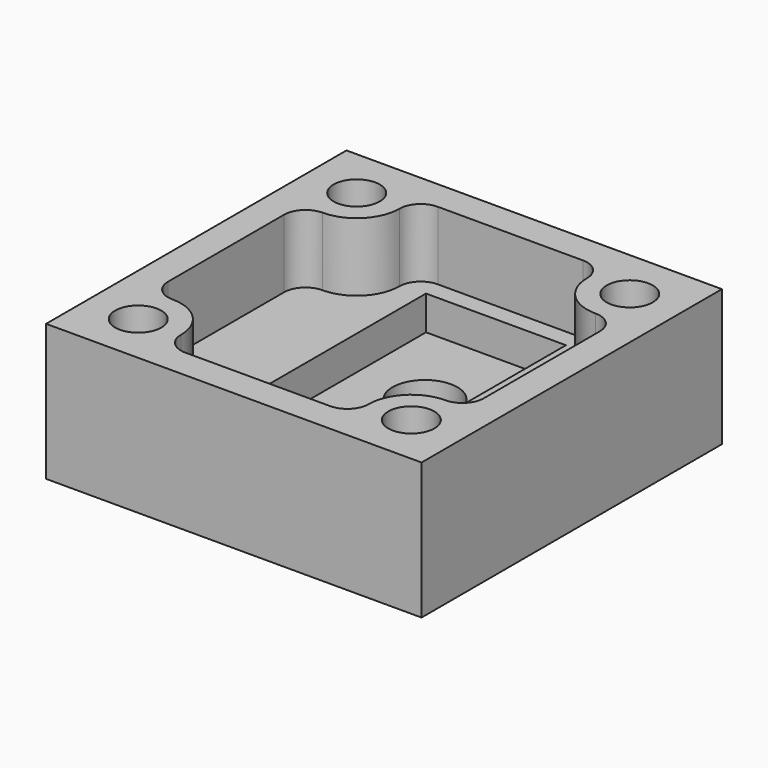
from build123d import *

# Parameters (mm, degrees)
F0_W     = 22
F0_H     = 22
F0_R     = 1.35
F0_R_2   = 1.9
F1_DEPTH = 8
F2_W     = 8.2
F2_H     = 16.4
F2_R     = 1.9
F3_DEPTH = 6
F4_DEPTH = 4
F5_R     = 1.24999


# Not quite as in the source:
# - a fillet or chamfer is up to 0.001 mm smaller than in the source, because OpenCascade refuses the exact size


with BuildPart() as f1:
    # F0 (on Top) → F1 (new body)
    with BuildSketch(Plane.XY):
        Rectangle(F0_W, F0_H)
        with Locations((-8, -8)):
            Circle(F0_R, mode=Mode.SUBTRACT)
        with Locations((8, -8)):
            Circle(F0_R, mode=Mode.SUBTRACT)
        with Locations((0, -3)):
            Circle(F0_R_2, mode=Mode.SUBTRACT)
        with Locations((-8, 8)):
            Circle(F0_R, mode=Mode.SUBTRACT)
        with Locations((0, 3)):
            Circle(F0_R_2, mode=Mode.SUBTRACT)
        with Locations((8, 8)):
            Circle(F0_R, mode=Mode.SUBTRACT)
    extrude(amount=F1_DEPTH)

    # F2 (on face) → F3 (cut)
    with BuildSketch(Plane.XY.offset(8)):
        Rectangle(F2_W, F2_H)
        with Locations((0, -3)):
            Circle(F2_R, mode=Mode.SUBTRACT)
        with Locations((0, 3)):
            Circle(F2_R, mode=Mode.SUBTRACT)
    extrude(amount=-F3_DEPTH, mode=Mode.SUBTRACT)

    # F2 (on face) → F4 (cut)
    with BuildSketch(Plane.XY.offset(8)):
        with BuildLine():
            ThreePointArc((-5.5, 8), (-6.232233047, 6.232233047), (-8, 5.5))
            Line((-8, 5.5), (-9.25, 5.5))
            Line((-9.25, 5.5), (-9.25, -5.5))
            Line((-9.25, -5.5), (-8, -5.5))
            ThreePointArc((-8, -5.5), (-6.232233047, -6.232233047), (-5.5, -8))
            Line((-5.5, -8), (-5.5, -9.25))
            Line((-5.5, -9.25), (5.5, -9.25))
            Line((5.5, -9.25), (5.5, -8))
            ThreePointArc((5.5, -8), (6.232233047, -6.232233047), (8, -5.5))
            Line((8, -5.5), (9.25, -5.5))
            Line((9.25, -5.5), (9.25, 5.5))
            Line((9.25, 5.5), (8, 5.5))
            ThreePointArc((8, 5.5), (6.232233047, 6.232233047), (5.5, 8))
            Line((5.5, 8), (5.5, 9.25))
            Line((5.5, 9.25), (-5.5, 9.25))
            Line((-5.5, 9.25), (-5.5, 8))
        make_face()
        Rectangle(F2_W, F2_H, mode=Mode.SUBTRACT)
    extrude(amount=-F4_DEPTH, mode=Mode.SUBTRACT)

    # F5 (radius 1.25 in the source; OpenCascade refuses exactly that, so slightly less here)
    f5_edges = [f1.edges().sort_by_distance(p)[0] for p in [
        (-9.25, 5.5, 6),
        (-5.5, 9.25, 6),
        (5.5, 9.25, 6),
        (9.25, 5.5, 6),
        (-9.25, -5.5, 6),
        (-5.5, -9.25, 6),
        (5.5, -9.25, 6),
        (9.25, -5.5, 6),
    ]]
    fillet(f5_edges, radius=F5_R)


solid = f1.part
